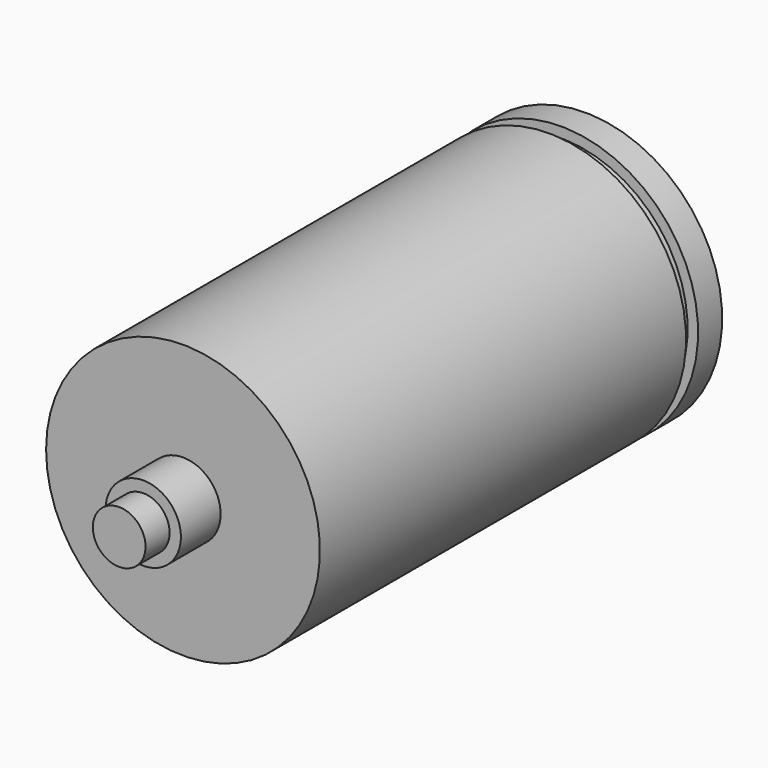
from build123d import *

# Parameters (mm, degrees)
F0_R      = 17.5
F1_DEPTH  = 20
F2_R      = 25
F2_R_2    = 17.5
F3_DEPTH  = 33
F4_R      = 90.957
F4_R_2    = 25
F5_DEPTH  = 304
F6_R      = 84
F7_DEPTH  = 10
F8_R      = 90.957
F8_R_2    = 84
F9_DEPTH  = 20
F10_R     = 25
F11_DEPTH = 33
F12_R     = 17.5
F13_DEPTH = 27
F14_R     = 15
F15_DEPTH = 30


with BuildPart() as f1:
    # F0 (on Front) → F1 (new body)
    with BuildSketch(Plane.XZ):
        Circle(F0_R)
    extrude(amount=-F1_DEPTH)

    # F2 (on face) → F3 (join)
    with BuildSketch(Plane(origin=(0, 20, 0), x_dir=(-1, 0, 0), z_dir=(0, 1, 0))):
        Circle(F2_R)
        Circle(F2_R_2, mode=Mode.SUBTRACT)
        Circle(F2_R_2)
    extrude(amount=F3_DEPTH)

    # F4 (on face) → F5 (join)
    with BuildSketch(Plane(origin=(0, 53, 0), x_dir=(-1, 0, 0), z_dir=(0, 1, 0))):
        Circle(F4_R)
        Circle(F4_R_2, mode=Mode.SUBTRACT)
        Circle(F4_R_2)
    extrude(amount=F5_DEPTH)

    # F10 (on face) → F11 (join)
    with BuildSketch(Plane(origin=(0, 357, 0), x_dir=(-1, 0, 0), z_dir=(0, 1, 0))):
        Circle(F10_R)
    extrude(amount=F11_DEPTH)

    # F12 (on face) → F13 (join)
    with BuildSketch(Plane(origin=(0, 390, 0), x_dir=(-1, 0, 0), z_dir=(0, 1, 0))):
        Circle(F12_R)
    extrude(amount=F13_DEPTH)

    # F14 (on face) → F15 (join)
    with BuildSketch(Plane(origin=(0, 417, 0), x_dir=(-1, 0, 0), z_dir=(0, 1, 0))):
        Circle(F14_R)
    extrude(amount=F15_DEPTH)


with BuildPart() as f7:
    # F6 (on face) → F7 (new body)
    with BuildSketch(Plane(origin=(0, 357, 0), x_dir=(-1, 0, 0), z_dir=(0, 1, 0))):
        Circle(F6_R)
    extrude(amount=F7_DEPTH)

    # F8 (on face) → F9 (join)
    with BuildSketch(Plane(origin=(0, 367, 0), x_dir=(-1, 0, 0), z_dir=(0, 1, 0))):
        Circle(F8_R)
        Circle(F8_R_2, mode=Mode.SUBTRACT)
        Circle(F8_R_2)
    extrude(amount=F9_DEPTH)


solid = Compound([f1.part, f7.part])
